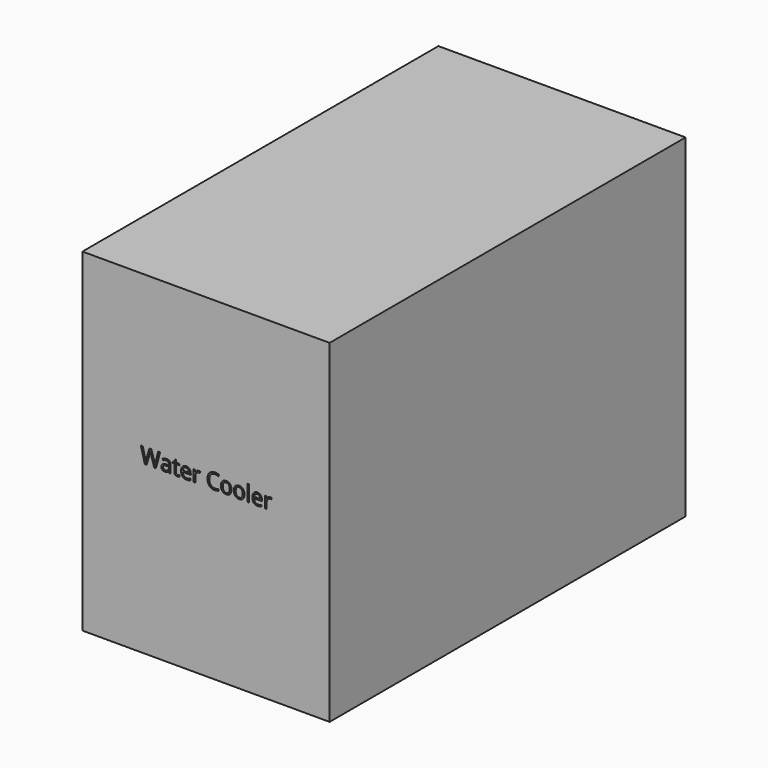
from build123d import *

# Parameters (mm, degrees)
F0_W         = 254
F0_H         = 342.9
F1_DEPTH     = 457.2
F2_TEXT_SIZE = 22.0381666217
F3_DEPTH     = 25.4


# Not quite as in the source:
# - Text() gives the source's letters only with a copy of the font that has no kerning and outlines rounded to 1/6400 em; it was checked with that copy


with BuildPart() as f1:
    # F0 (on Front) → F1 (new body)
    with BuildSketch(Plane.XZ):
        Rectangle(F0_W, F0_H)
    extrude(amount=-F1_DEPTH)

    # F2 (on face) → F3 (cut)
    with BuildSketch(Plane.XZ):
        with Locations((-67.322240506, 0)):
            Text('Water Cooler', F2_TEXT_SIZE, font='Open Sans', text_align=(TextAlign.LEFT, TextAlign.BOTTOM))
    extrude(amount=-F3_DEPTH, mode=Mode.SUBTRACT)


solid = f1.part
